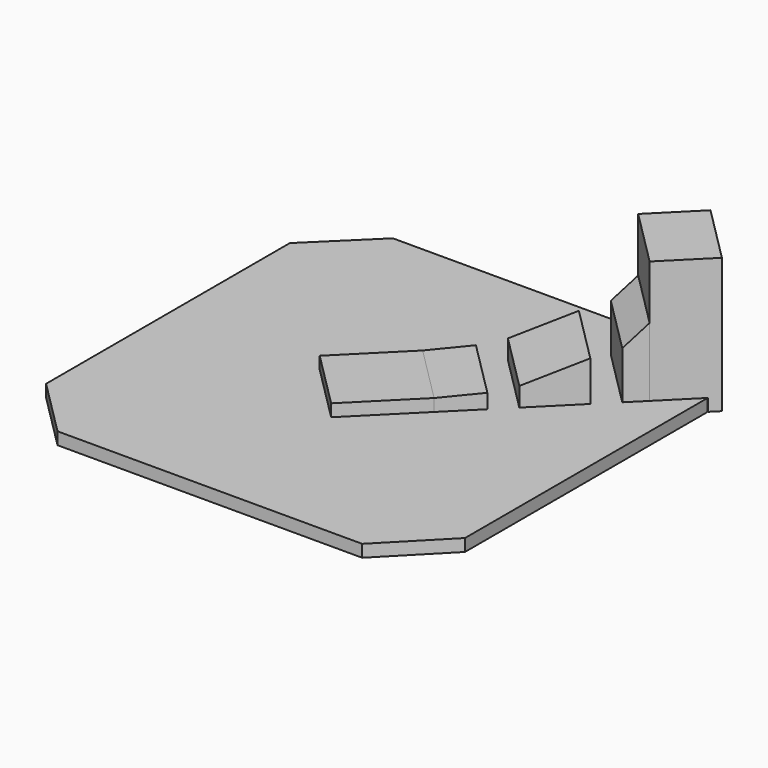
from build123d import *

# Parameters (mm, degrees)
F1_DEPTH  = 22
F3_DEPTH  = 22
F5_DEPTH  = 145
F6_DEPTH  = 145
F7_DEPTH  = 145
F8_DEPTH  = 145
F9_DEPTH  = 20
F11_DEPTH = 22


with BuildPart() as f1:
    # F0 (on Top) → F1 (new body)
    with BuildSketch(Plane.XY):
        Polygon((272.469516728, 375), (-271.380000358, 375), (-375, 273.5707356125), (-375, -272.469516728), (-272.469516728, -375), (273.5707356125, -375), (375, -271.380000358), (375, 272.469516728), align=None)
    extrude(amount=F1_DEPTH)

    # F2 (on face) → F3 (join)
    with BuildSketch(Plane.XY.offset(22)):
        Polygon((102.530483272, 0), (0, 102.5304832721), (-102.530483272, 0), (0, -102.530483272), align=None)
    extrude(amount=F3_DEPTH)


with BuildPart() as f5:
    # F4 (on face) → F5 (new body)
    with BuildSketch(Plane(origin=(51.265241636, -51.265241636, 0), x_dir=(0.7071067812, 0.7071067812, 0), z_dir=(0.7071067812, -0.7071067812, 0))):
        Polygon((72.5, 44), (72.5, 22), (147.5, 22), (147.5, 48), align=None)
    extrude(amount=-F5_DEPTH)


with BuildPart() as f6:
    # F4 (on face) → F6 (new body)
    with BuildSketch(Plane(origin=(51.265241636, -51.265241636, 0), x_dir=(0.7071067812, 0.7071067812, 0), z_dir=(0.7071067812, -0.7071067812, 0))):
        Polygon((192.5, 56.2), (192.5, 22), (292.5, 22), (292.5, 94), align=None)
    extrude(amount=-F6_DEPTH)


with BuildPart() as f7:
    # F4 (on face) → F7 (new body)
    with BuildSketch(Plane(origin=(51.265241636, -51.265241636, 0), x_dir=(0.7071067812, 0.7071067812, 0), z_dir=(0.7071067812, -0.7071067812, 0))):
        Polygon((337.5, 107.3), (337.5, 22), (376.0077297688, 22), (376.0077297688, 145), align=None)
    extrude(amount=-F7_DEPTH)


with BuildPart() as f8:
    # F4 (on face) → F8 (new body)
    with BuildSketch(Plane(origin=(51.265241636, -51.265241636, 0), x_dir=(0.7071067812, 0.7071067812, 0), z_dir=(0.7071067812, -0.7071067812, 0))):
        Polygon((376.0077297688, 145), (376.0077297688, 22), (457.8300858899, 22), (457.8300858899, 242), (376.0077297688, 242), align=None)
    extrude(amount=-F8_DEPTH)

    # F9 (add): a face of the model
    f9_faces = [f8.faces().sort_by_distance(p)[0] for p in [
        (323.734758364, 323.734758364, 132),
    ]]
    extrude(f9_faces, amount=F9_DEPTH)

    # F10 (on face) → F11 (join)
    with BuildSketch(Plane(origin=(0, 0, 22), x_dir=(1, 0, 0), z_dir=(0, 0, -1))):
        Polygon((272.7231215108, -375.2536047828), (286.6116523517, -389.1421356237), (389.1421356237, -286.6116523517), (375.2536047828, -272.7231215108), align=None)
    extrude(amount=F11_DEPTH)


solid = Compound([f1.part, f5.part, f6.part, f7.part, f8.part])
